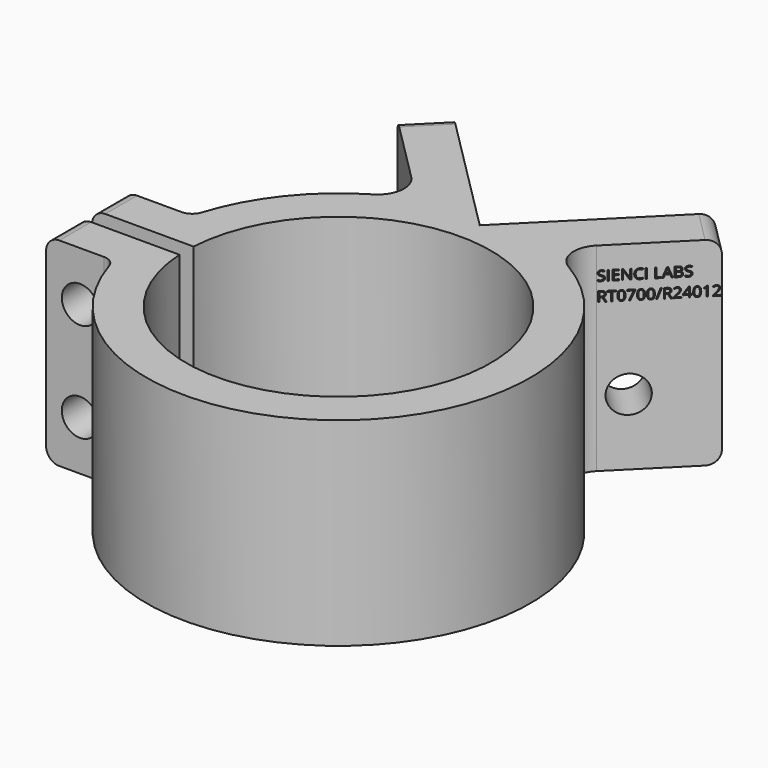
from build123d import *

# Parameters (mm, degrees)
F1_DEPTH      = 45
F2_R          = 4.125
F3_DEPTH      = 10
F4_R          = 4.125
F5_DEPTH      = 10
F6_R          = 4.125
F7_DEPTH      = 22
F8_R          = 3
F10_DEPTH     = 3
F11_R         = 6
F12_TEXT_SIZE = 3.0536622253
F13_DEPTH     = 0.5


# Not quite as in the source:
# - Text() gives the source's letters only with a copy of the font that has no kerning and outlines rounded to 1/6400 em; it was checked with that copy


with BuildPart() as f1:
    # F0 (on Top) → F1 (new body)
    with BuildSketch(Plane.XY):
        with BuildLine():
            Line((29.6984848098, 29.6984848098), (0, 0))
            Line((0, 0), (-29.6984848098, 29.6984848098))
            Line((-29.6984848098, 29.6984848098), (-36.7695526217, 22.627416998))
            Line((-36.7695526217, 22.627416998), (-14.9810608695, 0.8389252457))
            ThreePointArc((-14.9810608695, 0.8389252457), (-32.1987426867, -10.7512227709), (-42.086221023, -29))
            ThreePointArc((-42.086221023, -29), (-43.0061890439, -33.4641217943), (-43.4539986653, -38))
            Line((-43.4539986653, -38), (-34.4419801986, -38))
            ThreePointArc((-34.4419801986, -38), (34.5, -40), (-34.4419801986, -42))
            Line((-34.4419801986, -42), (-43.4539986653, -42))
            ThreePointArc((-43.4539986653, -42), (-43.0061890439, -46.5358782057), (-42.086221023, -51))
            ThreePointArc((-42.086221023, -51), (29.2487772291, -72.1987426867), (14.9810608695, 0.8389252457))
            Line((14.9810608695, 0.8389252457), (36.7695526217, 22.627416998))
            Line((36.7695526217, 22.627416998), (29.6984848098, 29.6984848098))
        make_face()
        with BuildLine():
            ThreePointArc((-43.4539986653, -38), (-43.0061890439, -33.4641217943), (-42.086221023, -29))
            Line((-42.086221023, -29), (-57.4539986653, -29))
            Line((-57.4539986653, -29), (-57.4539986653, -38))
            Line((-57.4539986653, -38), (-43.4539986653, -38))
        make_face()
        with BuildLine():
            Line((-57.4539986653, -51), (-42.086221023, -51))
            ThreePointArc((-42.086221023, -51), (-43.0061890439, -46.5358782057), (-43.4539986653, -42))
            Line((-43.4539986653, -42), (-57.4539986653, -42))
            Line((-57.4539986653, -42), (-57.4539986653, -51))
        make_face()
    extrude(amount=F1_DEPTH)

    # F2 (on face) → F3 (cut, through all)
    with BuildSketch(Plane(origin=(0, 0, 0), x_dir=(-0.7071067812, -0.7071067812, 0), z_dir=(-0.7071067812, 0.7071067812, 0))):
        with Locations((-25.4, 15)):
            Circle(F2_R)
    extrude(amount=-F3_DEPTH, mode=Mode.SUBTRACT)

    # F4 (on face) → F5 (cut, through all)
    with BuildSketch(Plane(origin=(0, 0, 0), x_dir=(-0.7071067812, 0.7071067812, 0), z_dir=(0.7071067812, 0.7071067812, 0))):
        with Locations((25.4, 15)):
            Circle(F4_R)
    extrude(amount=-F5_DEPTH, mode=Mode.SUBTRACT)

    # F6 (on face) → F7 (cut, through all)
    with BuildSketch(Plane.XZ.offset(51)):
        with Locations((-49.7701098441, 33.75)):
            Circle(F6_R)
        with Locations((-49.7701098441, 11.25)):
            Circle(F6_R)
    extrude(amount=-F7_DEPTH, mode=Mode.SUBTRACT)

    # F8
    f8_edges = [f1.edges().sort_by_distance(p)[0] for p in [
        (-57.453999, -33.5, 45),
        (-57.453999, -46.5, 45),
        (-57.453999, -46.5, 0),
        (-57.453999, -33.5, 0),
        (-33.234019, 26.162951, 45),
        (33.234019, 26.162951, 45),
        (33.234019, 26.162951, 0),
        (-33.234019, 26.162951, 0),
        (-42.086221, -29, 22.5),
        (-42.086221, -51, 22.5),
    ]]
    fillet(f8_edges, radius=F8_R)

    # F9 (on face) → F10 (cut)
    with BuildSketch(Plane(origin=(0, -29, 0), x_dir=(-1, 0, 0), z_dir=(0, 1, 0))):
        Polygon((56.6951098441, 37.7481506141), (49.7701098441, 41.7463012283), (42.8451098441, 37.7481506141), (42.8451098441, 29.7518493859), (49.7701098441, 25.7536987717), (56.6951098441, 29.7518493859), align=None)
        Polygon((56.6951098441, 7.2518493859), (56.6951098441, 15.2481506141), (49.7701098441, 19.2463012283), (42.8451098441, 15.2481506141), (42.8451098441, 7.2518493859), (49.7701098441, 3.2536987717), align=None)
    extrude(amount=-F10_DEPTH, mode=Mode.SUBTRACT)

    # F11
    f11_edges = [f1.edges().sort_by_distance(p)[0] for p in [
        (-14.981061, 0.838925, 22.5),
        (14.981061, 0.838925, 22.5),
    ]]
    fillet(f11_edges, radius=F11_R)

    # F12 (on face) → F13 (cut)
    with BuildSketch(Plane(origin=(7.0710678119, -7.0710678119, 0), x_dir=(0.7071067812, 0.7071067812, 0), z_dir=(0.7071067812, -0.7071067812, 0))):
        with Locations((19.6672321692, 37.8372258537)):
            Text('SIENCI LABS', F12_TEXT_SIZE, font='Open Sans', text_align=(TextAlign.LEFT, TextAlign.BOTTOM))
        with Locations((19.6672321692, 33.6842452273)):
            Text('RT0700/R24012', F12_TEXT_SIZE, font='Open Sans', text_align=(TextAlign.LEFT, TextAlign.BOTTOM))
    extrude(amount=-F13_DEPTH, mode=Mode.SUBTRACT)


solid = f1.part
